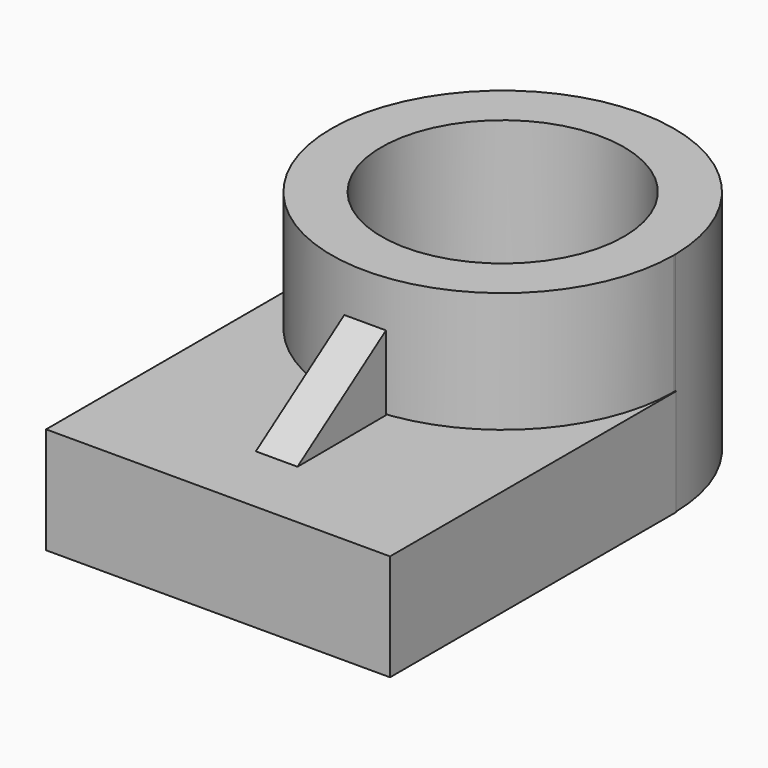
from build123d import *

# Parameters (mm, degrees)
F0_R     = 26.6037837969
F1_DEPTH = 49.784
F2_DEPTH = 23.368
F4_DEPTH = 4.572


# Not quite as in the source:
# - a feature names something its author has since deleted; it is built from what else it names


with BuildPart() as f1:
    # F0 (on Top) → F1 (new body)
    with BuildSketch(Plane.XY):
        with BuildLine():
            ThreePointArc((-37.5948276361, 39.2520837486), (-0.200781109, 1.2540912614), (37.5969721201, 38.8505272567))
            ThreePointArc((37.5969721201, 38.8505272567), (37.5964359953, 39.0513083657), (37.5948276361, 39.2520837486))
            ThreePointArc((37.5948276361, 39.2520837486), (0, 76.4474993769), (-37.5948276361, 39.2520837486))
        make_face()
        with Locations((0, 38.8505272567)):
            Circle(F0_R, mode=Mode.SUBTRACT)
    extrude(amount=F1_DEPTH)


with BuildPart() as f2:
    # F0 (on Top) → F2 (new body)
    with BuildSketch(Plane.XY):
        with BuildLine():
            ThreePointArc((37.5948276361, 39.2520837486), (37.5964359953, 39.0513083657), (37.5969721201, 38.8505272567))
            ThreePointArc((37.5969721201, 38.8505272567), (-0.200781109, 1.2540912614), (-37.5948276361, 39.2520837486))
            Line((-37.5948276361, 39.2520837486), (-37.7462469041, 39.2520837486))
            Line((-37.7462469041, 39.2520837486), (-37.7462469041, -39.2520837486))
            Line((-37.7462469041, -39.2520837486), (37.7462469041, -39.2520837486))
            Line((37.7462469041, -39.2520837486), (37.7462469041, 39.2520837486))
            Line((37.7462469041, 39.2520837486), (37.5948276361, 39.2520837486))
        make_face()
    extrude(amount=F2_DEPTH)

    # F3 (on Right) → F4 (join, symmetric)
    with BuildSketch(Plane.YZ):
        Polygon((-23.2066940516, 23.3460813761), (1.0955006583, 23.4599094838), (1.0955006583, 39.8510843515), align=None)
    extrude(amount=F4_DEPTH, both=True)


solid = Compound([f1.part, f2.part])
